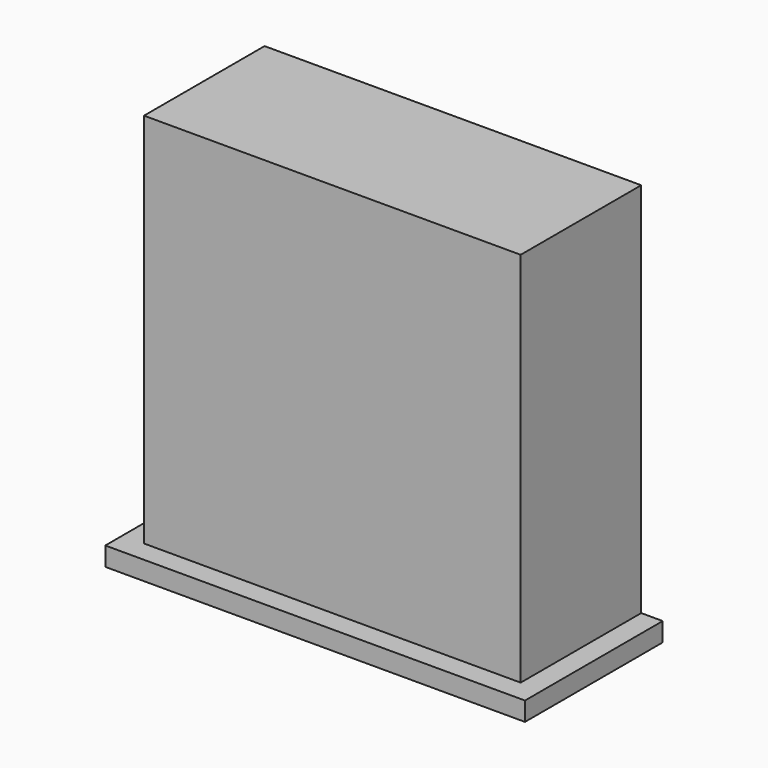
from build123d import *

# Parameters (mm, degrees)
F0_W         = 1778
F0_H         = 965.2
F1_DEPTH     = 1778
F2_TEXT_SIZE = 218.7096410327
F3_DEPTH     = 6.35
F4_DEPTH     = 254
F5_DEPTH     = 88.9
F6_W         = 1778
F6_H         = 88.9
F7_DEPTH     = 101.6
F9_DEPTH     = 101.6
F11_DEPTH    = 101.6


# Not quite as in the source:
# - Text() gives the source's letters only with a copy of the font that has no kerning and outlines rounded to 1/6400 em; it was checked with that copy


with BuildPart() as f1:
    # F0 (on Top) → F1 (new body)
    with BuildSketch(Plane.XY):
        with Locations((889, 482.6)):
            Rectangle(F0_W, F0_H)
    extrude(amount=F1_DEPTH)

    # F2 (on face) → F3 (join)
    with BuildSketch(Plane(origin=(0, 965.2, 0), x_dir=(-1, 0, 0), z_dir=(0, 1, 0))):
        with Locations((-1597.9287624359, 1507.4571371078)):
            Text('MAF-L-1.1', F2_TEXT_SIZE, font='Open Sans', text_align=(TextAlign.LEFT, TextAlign.BOTTOM))
    extrude(amount=F3_DEPTH)

    # F4 (cut): a face of the model
    f4_faces = [f1.faces().sort_by_distance(p)[0] for p in [
        (889, 0, 889),
    ]]
    extrude(f4_faces, amount=-F4_DEPTH, mode=Mode.SUBTRACT)

    # F5 (add): a face of the model
    f5_faces = [f1.faces().sort_by_distance(p)[0] for p in [
        (889, 609.6, 0),
    ]]
    extrude(f5_faces, amount=F5_DEPTH)

    # F6 (on face) → F7 (join)
    with BuildSketch(Plane.XZ.offset(-254)):
        with Locations((889, -44.45)):
            Rectangle(F6_W, F6_H)
    extrude(amount=F7_DEPTH)

    # F8 (on face) → F9 (join)
    with BuildSketch(Plane(origin=(0, 0, 0), x_dir=(0, -1, 0), z_dir=(-1, 0, 0))):
        Polygon((-152.4, -88.9), (-152.4, 0), (-254, 0), (-965.2, 0), (-965.2, -88.9), align=None)
    extrude(amount=F9_DEPTH)

    # F10 (on face) → F11 (join)
    with BuildSketch(Plane.YZ.offset(1778)):
        Polygon((254, 0), (152.4, 0), (152.4, -88.9), (965.2, -88.9), (965.2, 0), align=None)
    extrude(amount=F11_DEPTH)


solid = f1.part
